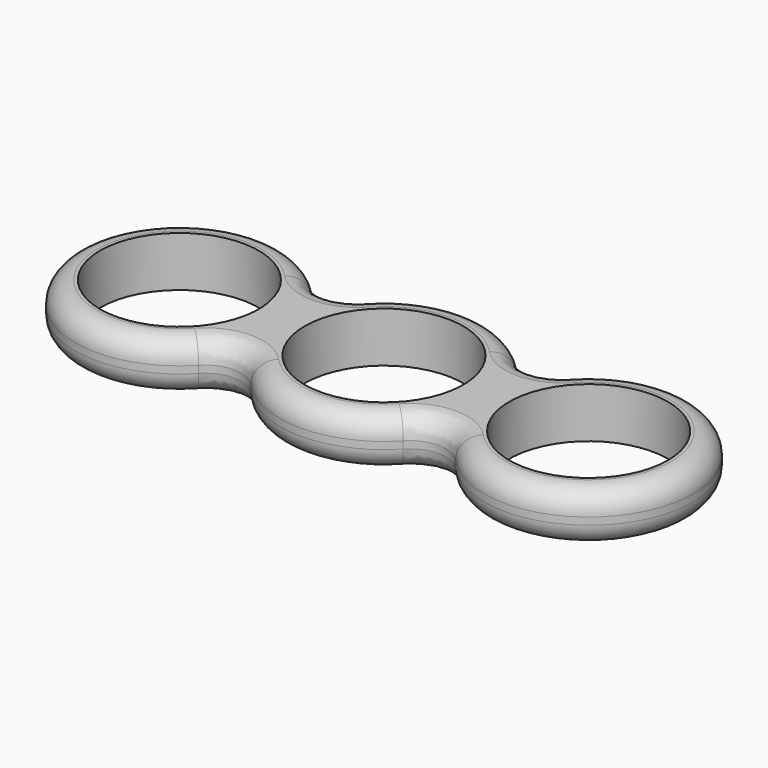
from build123d import *

# Parameters (mm, degrees)
F0_R     = 11.05
F1_DEPTH = 7
F2_R     = 5
F3_R     = 3


# Not quite as in the source:
# - a pattern or mirror of a feature is missing from the dataset's text; its kind, count and spacing are read off the source's solid
# - a feature names something its author has since deleted; it is built from what else it names


with BuildPart() as f1:
    # F0 (on Top) → F1 (new body)
    with BuildSketch(Plane.XY):
        with BuildLine():
            ThreePointArc((14.25, 2.6809513237), (14.437364718, 1.3462912018), (14.5, 0))
            ThreePointArc((14.5, 0), (14.437364718, -1.3462912018), (14.25, -2.6809513237))
            ThreePointArc((14.25, -2.6809513237), (29.8462912018, -14.437364718), (43, 0))
            ThreePointArc((43, 0), (29.8462912018, 14.437364718), (14.25, 2.6809513237))
        make_face()
        with Locations((28.5, 0)):
            Circle(F0_R, mode=Mode.SUBTRACT)
        with BuildLine():
            ThreePointArc((14.25, -2.6809513237), (14.437364718, -1.3462912018), (14.5, 0))
            ThreePointArc((14.5, 0), (14.437364718, 1.3462912018), (14.25, 2.6809513237))
            ThreePointArc((14.25, 2.6809513237), (14, 0), (14.25, -2.6809513237))
        make_face()
    extrude(amount=F1_DEPTH)


with BuildPart() as f1b:
    # F0 (on Top) → F1, piece 2 (new body)
    with BuildSketch(Plane.XY):
        with BuildLine():
            ThreePointArc((-14, 0), (-14.062635282, 1.3462912018), (-14.25, 2.6809513237))
            ThreePointArc((-14.25, 2.6809513237), (-14.5, 0), (-14.25, -2.6809513237))
            ThreePointArc((-14.25, -2.6809513237), (-14.062635282, -1.3462912018), (-14, 0))
        make_face()
    extrude(amount=F1_DEPTH)

    # F1_copies: F1 across plane
    add(f1.part.mirror(Plane(origin=(0, 0, 0), x_dir=(0, 0, -1), z_dir=(-1, 0, 0))))


with BuildPart() as f1_1:
    add(f1.part)

    add(f1b.part)  # F1_copies1 merges F1b
    # F1_copies1: F1 across plane
    add(f1.part.mirror(Plane(origin=(14.25, 0, 0), x_dir=(0, 0, -1), z_dir=(-1, 0, 0))))

    # F2
    f2_edges = [f1_1.edges().sort_by_distance(p)[0] for p in [
        (-14.25, -2.680951, 3.5),
        (14.25, -2.680951, 3.5),
        (14.25, 2.680951, 3.5),
        (-14.25, 2.680951, 3.5),
    ]]
    fillet(f2_edges, radius=F2_R)

    # F3
    f3_edges = [f1_1.edges().sort_by_distance(p)[0] for p in [
        (43, 0, 7),
        (43, 0, 0),
        (-43, 0, 0),
        (-43, 0, 7),
        (-14.25, 8.31118, 0),
        (-14.25, -8.31118, 0),
        (0, 14.5, 0),
        (0, -14.5, 0),
        (14.25, 8.31118, 0),
        (14.25, -8.31118, 0),
        (-14.25, 8.31118, 7),
        (-14.25, -8.31118, 7),
        (0, -14.5, 7),
        (0, 14.5, 7),
        (14.25, -8.31118, 7),
        (14.25, 8.31118, 7),
    ]]
    fillet(f3_edges, radius=F3_R)


solid = f1_1.part
